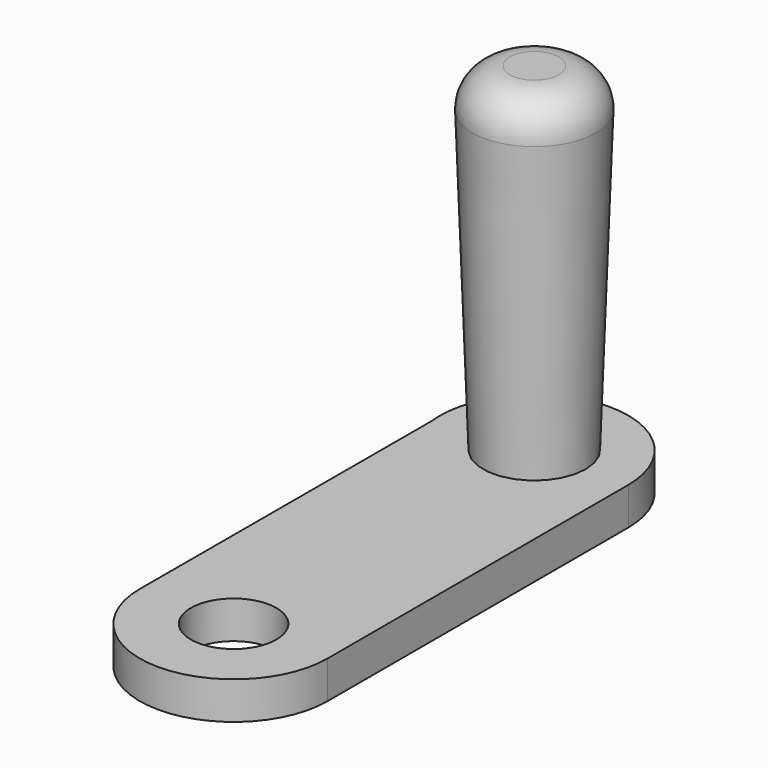
from build123d import *

# Parameters (mm, degrees)
F0_R     = 3.4141491506
F0_R_2   = 4
F1_DEPTH = 3
F2_DEPTH = 30
F2_TAPER = -2
F3_R     = 3


# Not quite as in the source:
# - ends of sketch curves that miss each other by under 0.0002 mm in the source are joined


with BuildPart() as f1:
    # F0 (on Top) → F1 (new body)
    with BuildSketch(Plane.XY):
        with BuildLine():
            ThreePointArc((7.5, 30), (0.4122865649, 37.488659412), (-7.4546719436, 30.8233263106))
            Line((-7.4546719436, 30.8233263106), (-7.4570616459, 29.1986064578))
            Line((-7.4570616459, 29.1986064578), (-7.4999918874, 0.0110312851))
            Line((-7.4999918874, 0.0110312851), (-7.5000081126, 0))
            ThreePointArc((-7.5000081126, 0), (4.0503e-06, -7.4944823293), (7.5, 0))
            Line((7.5, 0), (7.5, 30))
        make_face()
        Circle(F0_R, mode=Mode.SUBTRACT)
        with Locations((0, 30)):
            Circle(F0_R_2, mode=Mode.SUBTRACT)
        with BuildLine():
            Line((-7.4570616459, 29.1986064578), (-7.4546719436, 30.8233263106))
            ThreePointArc((-7.4546719436, 30.8233263106), (-7.4999918874, 30.0110312851), (-7.4570616459, 29.1986064578))
        make_face()
        with Locations((0, 30)):
            Circle(F0_R_2)
    extrude(amount=F1_DEPTH)


with BuildPart() as f2:
    # F0 (on Top) → F2 (new body)
    with BuildSketch(Plane.XY):
        with Locations((0, 30)):
            Circle(F0_R_2)
    extrude(amount=F2_DEPTH, taper=F2_TAPER)

    # F3
    f3_edges = [f2.edges().sort_by_distance(p)[0] for p in [
        (-5.047623, 30, 30),
    ]]
    fillet(f3_edges, radius=F3_R)


solid = Compound([f1.part, f2.part])
